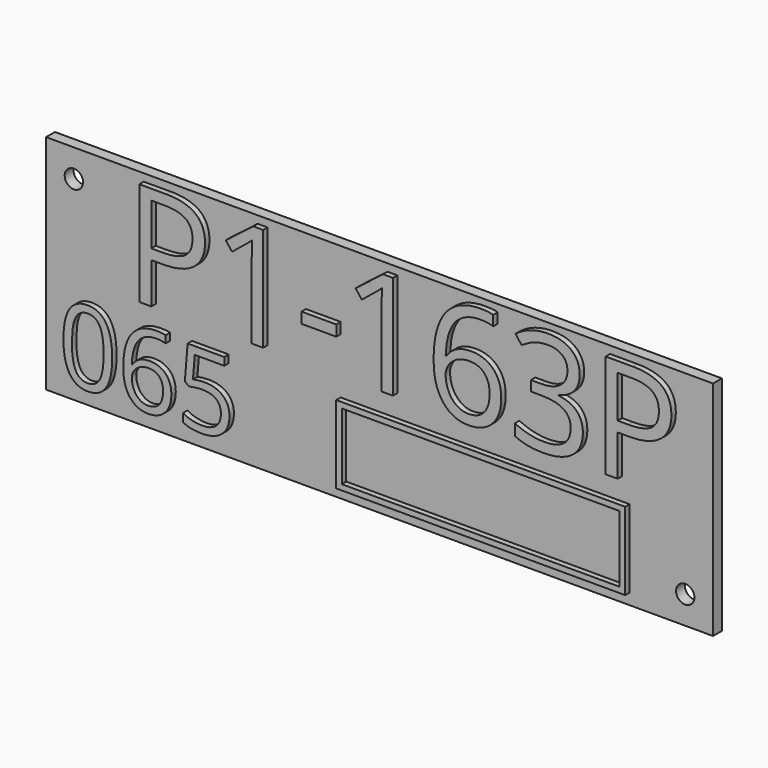
from build123d import *

# Parameters (mm, degrees)
F0_W         = 120
F0_H         = 40
F1_DEPTH     = 2
F3_D         = 3.3
F4_TEXT_SIZE = 26.1352499183
F5_DEPTH     = 1
F6_TEXT_SIZE = 18.5776487663
F7_DEPTH     = 1
F8_W         = 52
F8_H         = 14
F8_W_2       = 49.99999962
F8_H_2       = 11.99999962
F9_DEPTH     = 1


# Not quite as in the source:
# - Text() gives the source's letters only with a copy of the font that has no kerning and outlines rounded to 1/6400 em; it was checked with that copy


with BuildPart() as f1:
    # F0 (on Front) → F1 (new body)
    with BuildSketch(Plane.XZ):
        Rectangle(F0_W, F0_H)
    extrude(amount=F1_DEPTH)

    # F3 (through all)
    with Locations(Plane.XZ.offset(2)):
        with Locations((-55, 15), (55, -15)):
            Hole(F3_D / 2)

    # F4 (on face) → F5 (join)
    with BuildSketch(Plane.XZ.offset(2)):
        with Locations((-45, 0)):
            Text('P1-163P', F4_TEXT_SIZE, font='Open Sans', text_align=(TextAlign.LEFT, TextAlign.BOTTOM))
    extrude(amount=F5_DEPTH)

    # F6 (on face) → F7 (join)
    with BuildSketch(Plane.XZ.offset(2)):
        with Locations((-57, -17)):
            Text('065', F6_TEXT_SIZE, font='Open Sans', text_align=(TextAlign.LEFT, TextAlign.BOTTOM))
    extrude(amount=F7_DEPTH)

    # F8 (on face) → F9 (join)
    with BuildSketch(Plane.XZ.offset(2)):
        with Locations((19, -11)):
            Rectangle(F8_W, F8_H)
        with Locations((19, -11)):
            Rectangle(F8_W_2, F8_H_2, mode=Mode.SUBTRACT)
    extrude(amount=F9_DEPTH)


solid = f1.part
